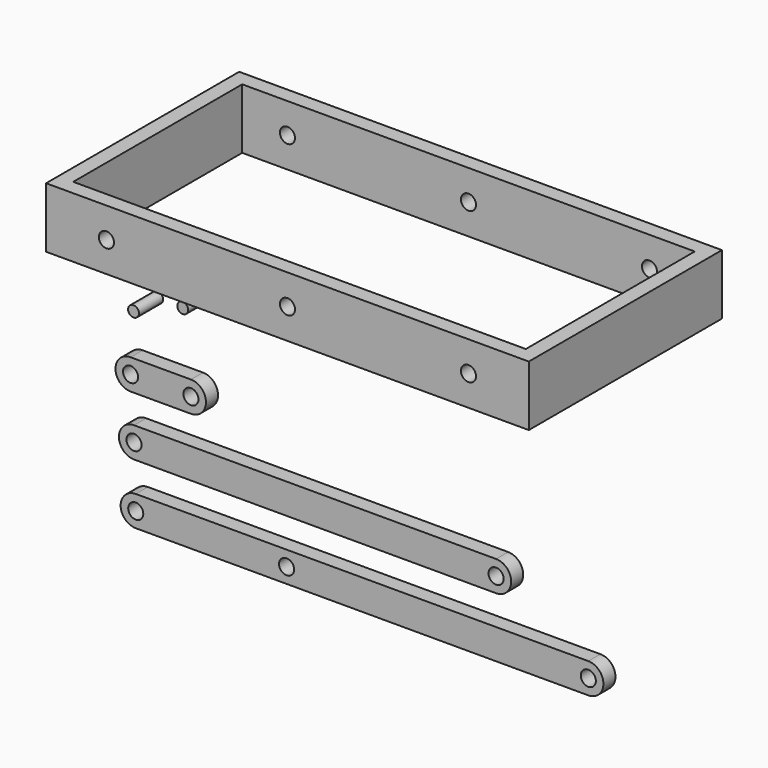
from build123d import *

# Parameters (mm, degrees)
F1_R      = 1.25
F2_DEPTH  = 2.5
F3_R      = 1.25
F4_DEPTH  = 2.5
F5_R      = 1.25
F6_DEPTH  = 2.5
F8_W      = 80
F8_H      = 40
F8_W_2    = 75
F8_H_2    = 35
F9_DEPTH  = 10
F10_R     = 1.25
F11_DEPTH = 40.001
F12_R     = 0.9
F13_DEPTH = 5
F14_R     = 0.9
F15_DEPTH = 7.5


with BuildPart() as f2:
    # F1 (on Front) → F2 (new body)
    with BuildSketch(Plane.XZ):
        with BuildLine():
            Line((10, 2.5), (0, 2.5))
            ThreePointArc((0, 2.5), (-2.5, 0), (0, -2.5))
            Line((0, -2.5), (10, -2.5))
            ThreePointArc((10, -2.5), (12.5, 0), (10, 2.5))
        make_face()
        Circle(F1_R, mode=Mode.SUBTRACT)
        with Locations((10, 0)):
            Circle(F1_R, mode=Mode.SUBTRACT)
    extrude(amount=F2_DEPTH)


with BuildPart() as f4:
    # F3 (on Front) → F4 (new body)
    with BuildSketch(Plane.XZ):
        with BuildLine():
            Line((60.5706622079, -7.232673876), (0.5706622079, -7.232673876))
            ThreePointArc((0.5706622079, -7.232673876), (-1.9293377921, -9.732673876), (0.5706622079, -12.232673876))
            Line((0.5706622079, -12.232673876), (60.5706622079, -12.232673876))
            ThreePointArc((60.5706622079, -12.232673876), (63.0706622079, -9.732673876), (60.5706622079, -7.232673876))
        make_face()
        with Locations((0.5706622079, -9.732673876)):
            Circle(F3_R, mode=Mode.SUBTRACT)
        with Locations((60.5706622079, -9.732673876)):
            Circle(F3_R, mode=Mode.SUBTRACT)
    extrude(amount=F4_DEPTH)


with BuildPart() as f6:
    # F5 (on Front) → F6 (new body)
    with BuildSketch(Plane.XZ):
        with BuildLine():
            Line((75.8570737601, -17.1626018733), (0.8570737601, -17.1626018733))
            ThreePointArc((0.8570737601, -17.1626018733), (-1.6429262399, -19.6626018733), (0.8570737601, -22.1626018733))
            Line((0.8570737601, -22.1626018733), (75.8570737601, -22.1626018733))
            ThreePointArc((75.8570737601, -22.1626018733), (78.3570737601, -19.6626018733), (75.8570737601, -17.1626018733))
        make_face()
        with Locations((0.8570737601, -19.6626018733)):
            Circle(F5_R, mode=Mode.SUBTRACT)
        with Locations((25.8570737601, -19.6626018733)):
            Circle(F5_R, mode=Mode.SUBTRACT)
        with Locations((75.8570737601, -19.6626018733)):
            Circle(F5_R, mode=Mode.SUBTRACT)
    extrude(amount=F6_DEPTH)


with BuildPart() as f9:
    # F8 (on offset) → F9 (new body)
    with BuildSketch(Plane.XY.offset(25)):
        with Locations((40, 0)):
            Rectangle(F8_W, F8_H)
        with Locations((40, 0)):
            Rectangle(F8_W_2, F8_H_2, mode=Mode.SUBTRACT)
    extrude(amount=F9_DEPTH)

    # F10 (on face) → F11 (cut, through all)
    with BuildSketch(Plane.XZ.offset(20)):
        with Locations((10, 30)):
            Circle(F10_R)
        with Locations((70, 30)):
            Circle(F10_R)
        with Locations((40, 30)):
            Circle(F10_R)
    extrude(amount=-F11_DEPTH, mode=Mode.SUBTRACT)


with BuildPart() as f13:
    # F12 (on Front) → F13 (new body)
    with BuildSketch(Plane.XZ):
        with Locations((2.488047583, 11.0218990594)):
            Circle(F12_R)
    extrude(amount=F13_DEPTH)


with BuildPart() as f15:
    # F14 (on Front) → F15 (new body)
    with BuildSketch(Plane.XZ):
        with Locations((12.6421162859, 15.8389676362)):
            Circle(F14_R)
    extrude(amount=F15_DEPTH)


solid = Compound([f2.part, f4.part, f6.part, f9.part, f13.part, f15.part])
